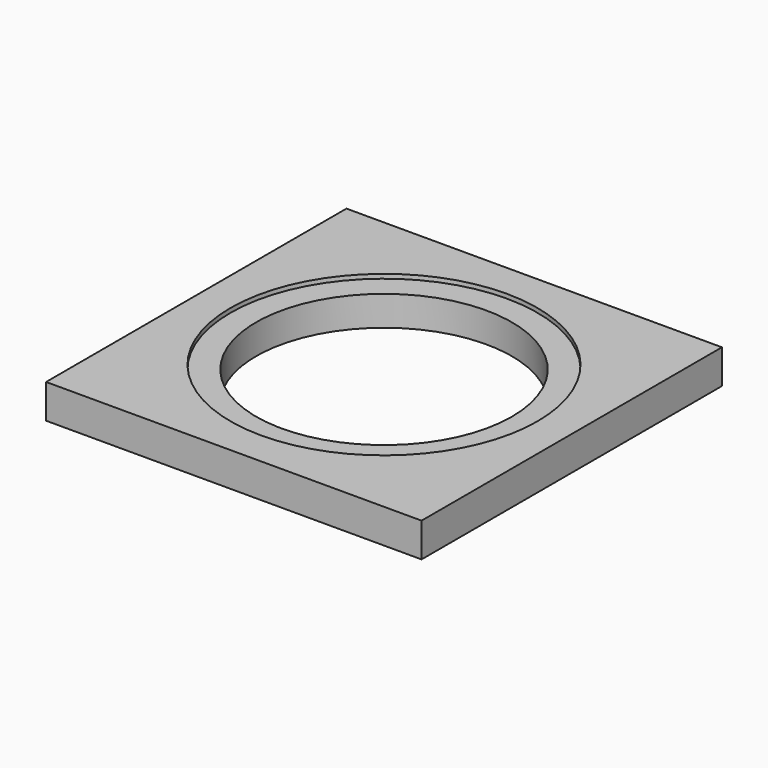
from build123d import *

# Parameters (mm, degrees)
F0_W     = 279.4
F0_H     = 279.4
F1_DEPTH = 25.4
F2_R     = 114.2111
F3_DEPTH = 3.175
F4_R     = 95.1611
F5_DEPTH = 22.225


# Not quite as in the source:
# - a feature of the source that left no trace in its solid (it failed there, or was rolled back) is left out


with BuildPart() as f1:
    # F0 (on Top) → F1 (new body)
    with BuildSketch(Plane.XY):
        Rectangle(F0_W, F0_H)
    extrude(amount=F1_DEPTH)

    # F2 (on face) → F3 (cut)
    with BuildSketch(Plane.XY.offset(25.4)):
        Circle(F2_R)
    extrude(amount=-F3_DEPTH, mode=Mode.SUBTRACT)

    # F4 (on face) → F5 (cut)
    with BuildSketch(Plane.XY.offset(22.225)):
        Circle(F4_R)
    extrude(amount=-F5_DEPTH, mode=Mode.SUBTRACT)


solid = f1.part
